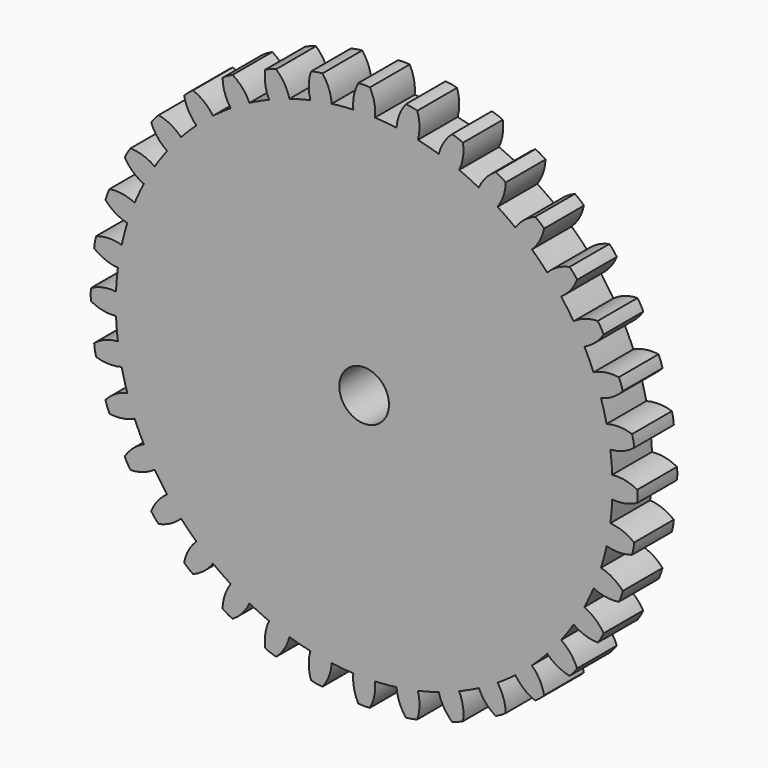
from build123d import *

# Parameters (mm, degrees)
F0_R     = 2.5
F1_DEPTH = 5
F2_COUNT = 36


with BuildPart() as f1:
    # F0 (on Front) → F1 (new body)
    with BuildSketch(Plane.XZ):
        with BuildLine():
            ThreePointArc((-1.0904846841, 24.9762055395), (-17.2878263946, -18.0590990515), (25, 0))
            ThreePointArc((25, 0), (18.0590990515, 17.2878263946), (1.0904846841, 24.9762055395))
            ThreePointArc((1.0904846841, 24.9762055395), (0, 25), (-1.0904846841, 24.9762055395))
        make_face()
        Circle(F0_R, mode=Mode.SUBTRACT)
        with BuildLine():
            ThreePointArc((-1.0904846841, 24.9762055395), (0, 25), (1.0904846841, 24.9762055395))
            ThreePointArc((1.0904846841, 24.9762055395), (1.0282240972, 26.2730263905), (0.5861298281, 27.49375296))
            ThreePointArc((0.5861298281, 27.49375296), (0, 27.5257167689), (-0.5861298281, 27.49375296))
            ThreePointArc((-0.5861298281, 27.49375296), (-1.0282240972, 26.2730263905), (-1.0904846841, 24.9762055395))
        make_face()
    extrude(amount=F1_DEPTH)

    # F2: F1 ×36 about axis
    f2_axis = Axis((0, 0, 0), (0, 1, 0))


with BuildPart() as f1_1:
    add(f1.part)
    for i in range(1, F2_COUNT):
        add(f1.part.rotate(f2_axis, i * 360 / F2_COUNT))


solid = f1_1.part
